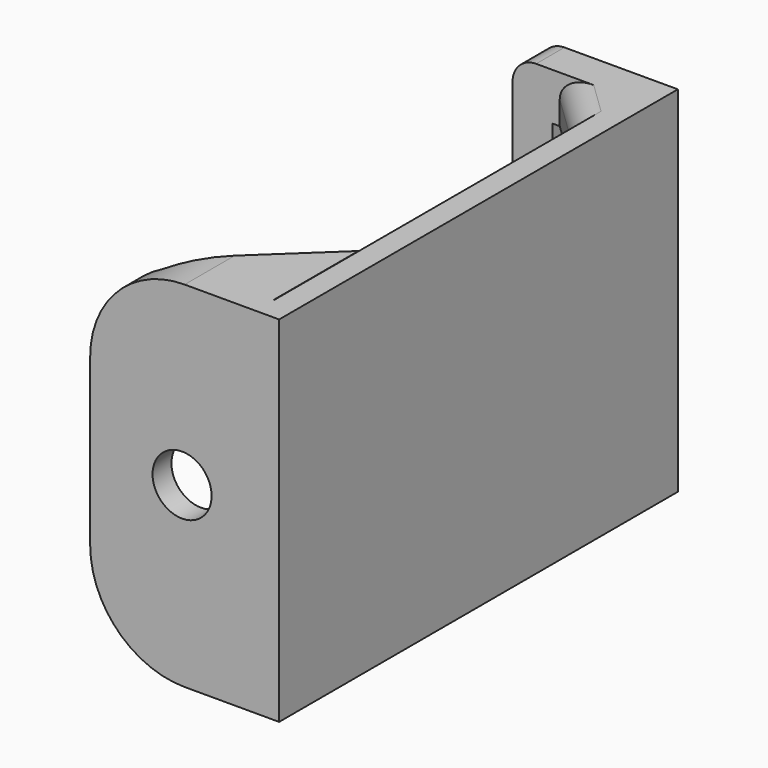
from build123d import *

# Parameters (mm, degrees)
F1_E1_W   = 20.1
F1_E1_H   = 15
F2_DEPTH  = 1
F1_E0_W   = 8
F1_E0_H   = 15
F3_DEPTH  = 1
F5_DEPTH  = 1
F7_DEPTH  = 1
F9_DEPTH  = 1.5
F11_R     = 4
F12_R     = 1
F13_SIZE2 = 2.7039285695
F13_SIZE  = 2.8
F14_R     = 1
F16_D     = 2.5
F16_DEPTH = 3
F16_TIP   = 0.7510757738


with BuildPart() as f2:
    # F1_E1 (on explicit) → F2 (new body)
    with BuildSketch(Plane.YZ):
        with Locations((10.05, 7.5)):
            Rectangle(F1_E1_W, F1_E1_H)
    extrude(amount=-F2_DEPTH)

    # F1_E0 (on explicit) → F3 (join)
    with BuildSketch(Plane(origin=(-8, 0, 0), x_dir=(1, 0, 0), z_dir=(0, -1, 0))):
        with Locations((4, 7.5)):
            Rectangle(F1_E0_W, F1_E0_H)
    extrude(amount=F3_DEPTH)

    # F4 (on Top) → F5 (join)
    with BuildSketch(Plane.XY):
        Polygon((-5.7501993142, 0), (-1.0129548609, 0), (-1.0129548609, 4.4631827623), align=None)
    extrude(amount=F5_DEPTH)

    # F6 (on face) → F7 (join)
    with BuildSketch(Plane.XY.offset(15)):
        Polygon((-5.7530710474, 0), (-1.0158265941, 0), (-1.0158265941, 4.4631827623), align=None)
    extrude(amount=-F7_DEPTH)

    # F8 (on face) → F9 (join)
    with BuildSketch(Plane(origin=(0, 20.1, 0), x_dir=(-1, 0, 0), z_dir=(0, 1, 0))):
        Polygon((5.8, 15), (0, 15), (0, 13), (4.1, 13), (4.1, 2), (0, 2), (0, 0), (5.8, 0), align=None)
    extrude(amount=-F9_DEPTH)

    # F10: union 

    # F11
    f11_edges = [f2.edges().sort_by_distance(p)[0] for p in [
        (-8, -0.5, 0),
        (-8, -0.5, 15),
    ]]
    fillet(f11_edges, radius=F11_R)

    # F12
    f12_edges = [f2.edges().sort_by_distance(p)[0] for p in [
        (-5.8, 19.35, 0),
        (-5.8, 19.35, 15),
    ]]
    fillet(f12_edges, radius=F12_R)

    # F13
    f13_edges = [f2.edges().sort_by_distance(p)[0] for p in [
        (-1, 18.6, 1),
        (-1, 18.6, 14),
    ]]
    chamfer(f13_edges, length=F13_SIZE, length2=F13_SIZE2)

    # F14
    f14_edges = [f2.edges().sort_by_distance(p)[0] for p in [
        (-2.4, 17.248036, 0),
        (-2.4, 17.248036, 15),
    ]]
    fillet(f14_edges, radius=F14_R)

    # F16
    with Locations(Plane.XZ.offset(1)):
        with Locations((-4.1083735414, 7.4923457578)):
            Hole(F16_D / 2, depth=F16_DEPTH)
            with Locations((0, 0, -(F16_DEPTH + F16_TIP / 2))):  # 118° drill point
                Cone(0, F16_D / 2, F16_TIP, mode=Mode.SUBTRACT)


solid = f2.part
